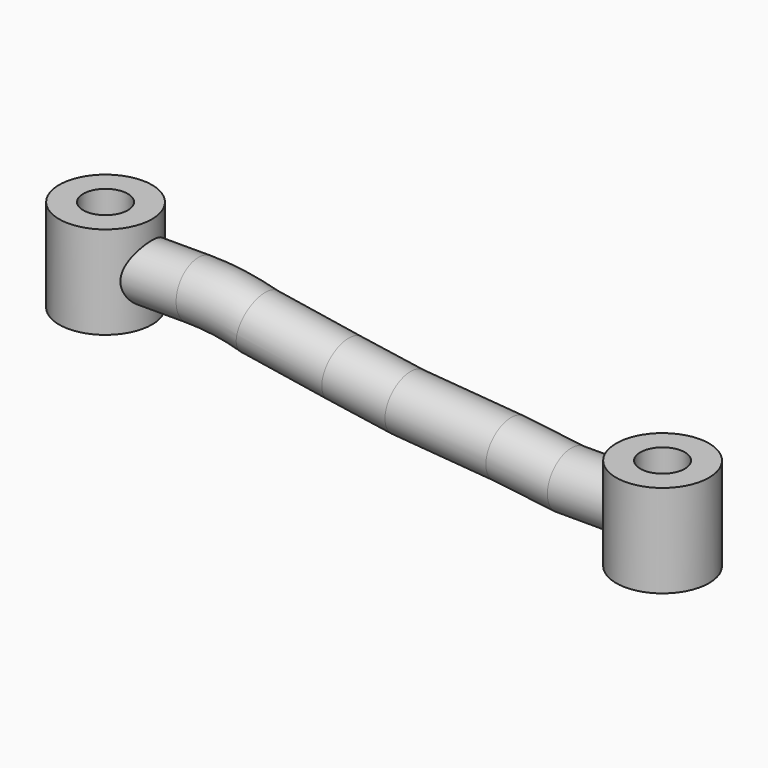
from build123d import *

# Parameters (mm, degrees)
F0_R      = 12.5
F0_R_2    = 6
F1_DEPTH  = 25
F3_R      = 12.5
F3_R_2    = 6
F4_DEPTH  = 12.5
F5_R      = 7.5
F7_R      = 6
F8_DEPTH  = 25
F9_R      = 6
F10_DEPTH = 25


# Not quite as in the source:
# - a feature names something its author has since deleted; it is built from what else it names


with BuildPart() as f1:
    # F0 (on Top) → F1 (new body)
    with BuildSketch(Plane.XY):
        Circle(F0_R)
        Circle(F0_R_2, mode=Mode.SUBTRACT)
    extrude(amount=F1_DEPTH)



with BuildPart() as f4:
    # F3 (on Top) → F4 (new body, symmetric)
    with BuildSketch(Plane.XY):
        with Locations((150, 0)):
            Circle(F3_R)
        with Locations((150, 0)):
            Circle(F3_R_2, mode=Mode.SUBTRACT)
    extrude(amount=F4_DEPTH, both=True)


with BuildPart() as f1_1:
    add(f1.part)

    add(f4.part)  # F6 merges F4
    # F6: sweep along a path in F2
    with BuildLine(Plane.XZ) as f6_path:
        Line((0, 12.5), (25, 12.5))
        ThreePointArc((25, 12.5), (33.2790451747, 11.9260667636), (41.399703043, 10.2152470332))
        Line((41.399703043, 10.2152470332), (64.3324330449, 6.6001820378))
        Line((64.3324330449, 6.6001820378), (81.3044384122, 4.0990444832))
        Line((81.3044384122, 4.0990444832), (108.4596440196, 1.9552123267))
        Line((108.4596440196, 1.9552123267), (125, 0))
        Line((125, 0), (150, 0))
    # F5 (on Right) → F6 (sweep)
    with BuildSketch(Plane.YZ):
        with Locations((0, 12.5)):
            Circle(F5_R)
    sweep(path=f6_path.line, transition=Transition.RIGHT)

    # F7 (on Top) → F8 (cut)
    with BuildSketch(Plane.XY):
        Circle(F7_R)
    extrude(amount=F8_DEPTH, mode=Mode.SUBTRACT)

    # F9 (on face) → F10 (cut)
    with BuildSketch(Plane.XY.offset(12.5)):
        with Locations((150, 0)):
            Circle(F9_R)
    extrude(amount=-F10_DEPTH, mode=Mode.SUBTRACT)


solid = f1_1.part
